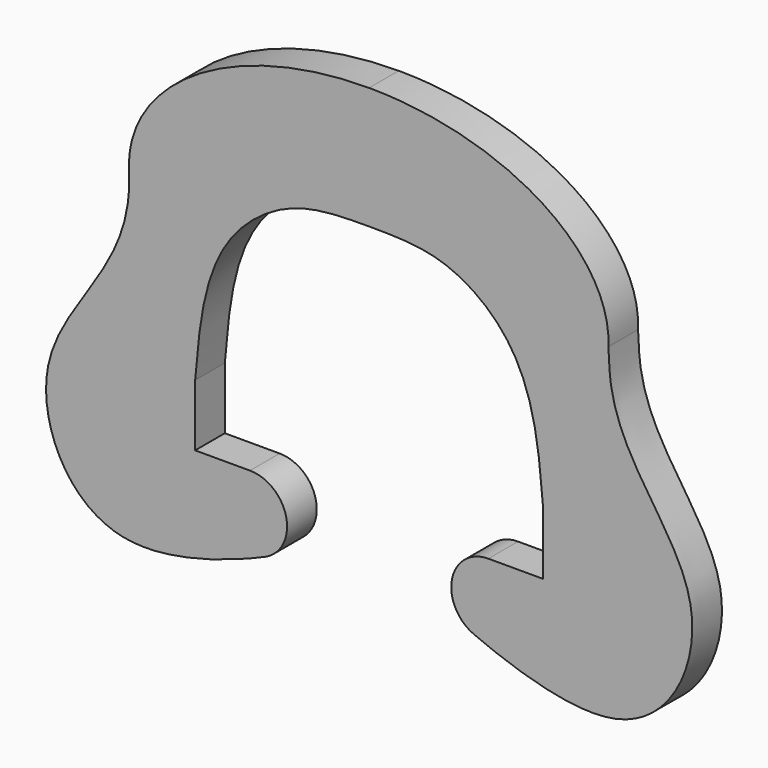
from build123d import *

# Parameters (mm, degrees)
F1_DEPTH = 3


# Not quite as in the source:
# - ends of sketch curves that miss each other by under 0.0002 mm in the source are joined
# - the dataset's text gives a spline's control points without its knots; the knots are read off the source's solid


with BuildPart() as f1:
    # F0 (on Front) → F1 (new body)
    with BuildSketch(Plane.XZ):
        with BuildLine():
            Line((-9.636137, -11.080088), (-14.07, -11.080088))
            Line((-14.07, -11.080088), (-14.07, -6.080088))
            add(Edge.make_bspline(
                [(-14.07, -6.080088), (-13.725678, -2.009613), (-13.197272, 4.237053), (-6.222695, 9.414593), (-2.060159, 9.423293), (0, 9.427599)],
                knots=[0, 0, 0, 0, 11.597106, 17.797245, 23.872878, 23.872878, 23.872878, 23.872878], degree=3))
            add(Edge.make_bspline(
                [(14.07, -6.080088), (13.725679, -2.009613), (13.197273, 4.237053), (6.222696, 9.414593), (2.06016, 9.423293), (0, 9.427599)],
                knots=[0, 0, 0, 0, 11.597106, 17.797245, 23.872878, 23.872878, 23.872878, 23.872878], degree=3))
            Line((14.07, -6.080088), (14.07, -11.080088))
            Line((14.07, -11.080088), (9.636138, -11.080088))
            ThreePointArc((9.636138, -11.080088), (6.6980962866, -13.4735314153), (8.4480789685, -16.8348140731))
            add(Edge.make_bspline(
                [(19.339969, 7.161527), (19.387769, 6.678303), (19.412006, -0.419852), (29.48044, -7.102045), (22.588634, -22.151196), (11.198451, -18.020996), (8.4480789685, -16.8348140731)],
                knots=[26.688985, 26.688985, 26.688985, 26.688985, 28.557776, 42.872008, 54.1154, 62.665306, 62.665306, 62.665306, 62.665306], degree=3))
            add(Edge.make_bspline(
                [(19.339969, 7.161527), (19.9265814181, 19.2748150047), (-0.0078359998, 19.2919222589)],
                knots=[6.253754, 6.253754, 6.253754, 7.8525699735, 7.8525699735, 7.8525699735], degree=2, weights=[1, 0.6971312715, 1]))
            add(Edge.make_bspline(
                [(-0.008117, 19.291903), (-0.008023, 19.291909), (-0.007929, 19.291915), (-0.0078359998, 19.2919222589)],
                knots=[0, 0, 0, 0, 1, 1, 1, 1], degree=3))
            add(Edge.make_bspline(
                [(-0.008117, 19.291903), (-0.008221, 19.291909), (-0.008326, 19.291916), (-0.008431, 19.291922)],
                knots=[0, 0, 0, 0, 1, 1, 1, 1], degree=3))
            add(Edge.make_bspline(
                [(-0.008431, 19.291922), (-20.136683318, 19.3088207532), (-19.4059855754, 7.0805132175)],
                knots=[1.5694153625, 1.5694153625, 1.5694153625, 3.1779026928, 3.1779026928, 3.1779026928], degree=2, weights=[1, 0.693656226, 1]))
            add(Edge.make_bspline(
                [(-19.4059855754, 7.0805132175), (-19.387768, 6.678303), (-19.412005, -0.419852), (-29.48044, -7.102045), (-22.588633, -22.151196), (-11.19845, -18.020996), (-8.448078, -16.834814)],
                knots=[26.688985, 26.688985, 26.688985, 26.688985, 28.557776, 42.872008, 54.1154, 62.665306, 62.665306, 62.665306, 62.665306], degree=3))
            ThreePointArc((-8.448078, -16.834814), (-6.6980952866, -13.4735314153), (-9.636137, -11.080088))
        make_face()
    extrude(amount=F1_DEPTH)


solid = f1.part
